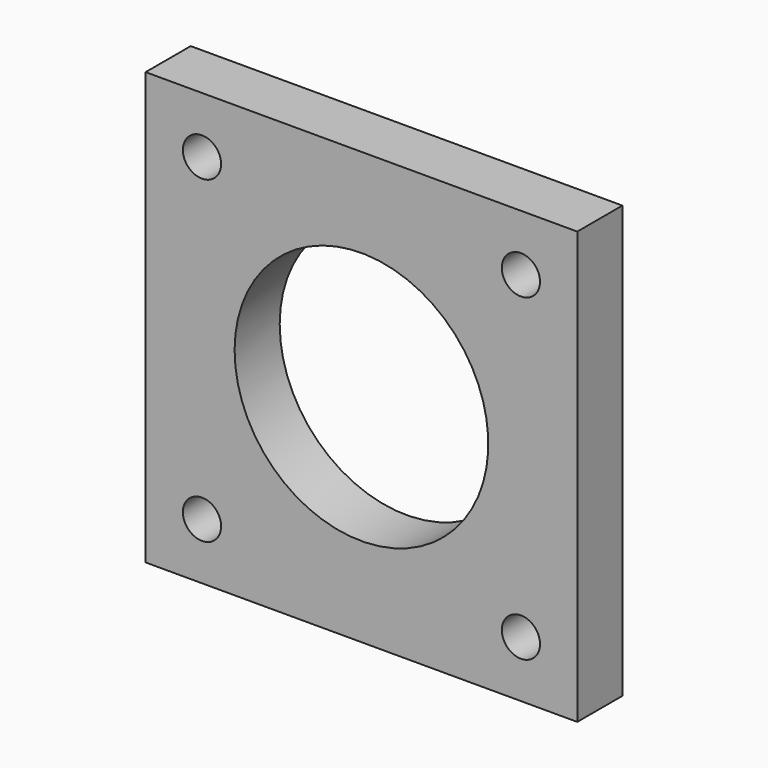
from build123d import *

# Parameters (mm, degrees)
F0_W      = 48.6210244843
F0_H      = 48.6210244843
F0_R      = 2.15265
F1_DEPTH  = 6.35
F6_W      = 2.794
F6_H      = 1.27
F8_R      = 0.2032
F9_R      = 14.2875
F10_DEPTH = 6.351


with BuildPart() as f1:
    # F0 (on Front) → F1 (new body)
    with BuildSketch(Plane.XZ):
        Rectangle(F0_W, F0_H)
        with Locations((-17.9605122421, -17.9605122421)):
            Circle(F0_R, mode=Mode.SUBTRACT)
        with Locations((17.9605122421, -17.9605122421)):
            Circle(F0_R, mode=Mode.SUBTRACT)
        with Locations((-17.9605122421, 17.9605122421)):
            Circle(F0_R, mode=Mode.SUBTRACT)
        with Locations((17.9605122421, 17.9605122421)):
            Circle(F0_R, mode=Mode.SUBTRACT)
    extrude(amount=F1_DEPTH)

    # F6 (on 3pt) → F7 (revolve, cut)
    with BuildSketch(Plane(origin=(0, 0, 0), x_dir=(1, 0, 0), z_dir=(0, 0, -1))):
        with Locations((-19.7993, 0.635)):
            Rectangle(F6_W, F6_H)
    revolve(axis=Axis((0, 0.4501026124, 0), (0, -1, 0)), mode=Mode.SUBTRACT)

    # F8
    f8_edges = [f1.edges().sort_by_distance(p)[0] for p in [
        (21.1963, -1.27, 0),
        (18.4023, 0, 0),
    ]]
    fillet(f8_edges, radius=F8_R)

    # F9 (on face) → F10 (cut, through all)
    with BuildSketch(Plane(origin=(0, 0, 0), x_dir=(-1, 0, 0), z_dir=(0, 1, 0))):
        Circle(F9_R)
    extrude(amount=-F10_DEPTH, mode=Mode.SUBTRACT)


solid = f1.part
